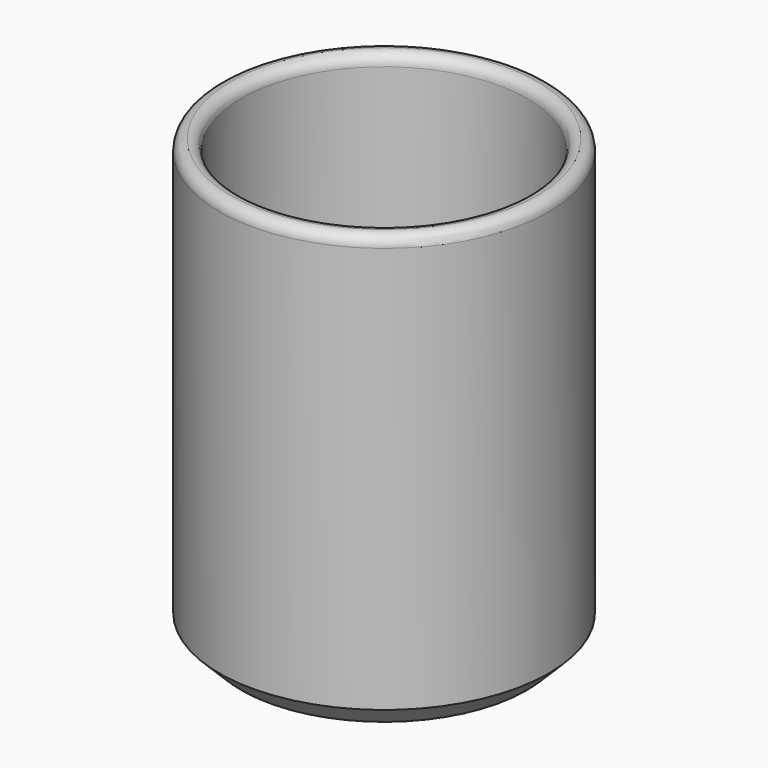
from build123d import *

# Parameters (mm, degrees)
F0_R     = 38.1
F1_DEPTH = 101.6
F2_T     = -5.08
F3_R     = 7.62
F4_R     = 2.53999
F5_SIZE  = 5.08


# Not quite as in the source:
# - a fillet or chamfer is up to 0.001 mm smaller than in the source, because OpenCascade refuses the exact size


with BuildPart() as f1:
    # F0 (on Top) → F1 (new body)
    with BuildSketch(Plane.XY):
        with Locations((-51.5342205763, 6.2507814728)):
            Circle(F0_R)
    extrude(amount=F1_DEPTH)

    # F2
    f2_openings = [f1.faces().sort_by_distance(p)[0] for p in [
        (-51.534221, 6.250781, 101.6),
    ]]
    offset(amount=F2_T, openings=f2_openings)

    # F3
    f3_edges = [f1.edges().sort_by_distance(p)[0] for p in [
        (-84.554221, 6.250781, 5.08),
    ]]
    fillet(f3_edges, radius=F3_R)

    # F4 (radius 2.54 in the source; OpenCascade refuses exactly that, so slightly less here)
    f4_edges = [f1.edges().sort_by_distance(p)[0] for p in [
        (-84.554221, 6.250781, 101.6),
        (-89.634221, 6.250781, 101.6),
    ]]
    fillet(f4_edges, radius=F4_R)

    # F5
    f5_edges = [f1.edges().sort_by_distance(p)[0] for p in [
        (-89.634221, 6.250781, 0),
    ]]
    chamfer(f5_edges, length=F5_SIZE)


solid = f1.part
